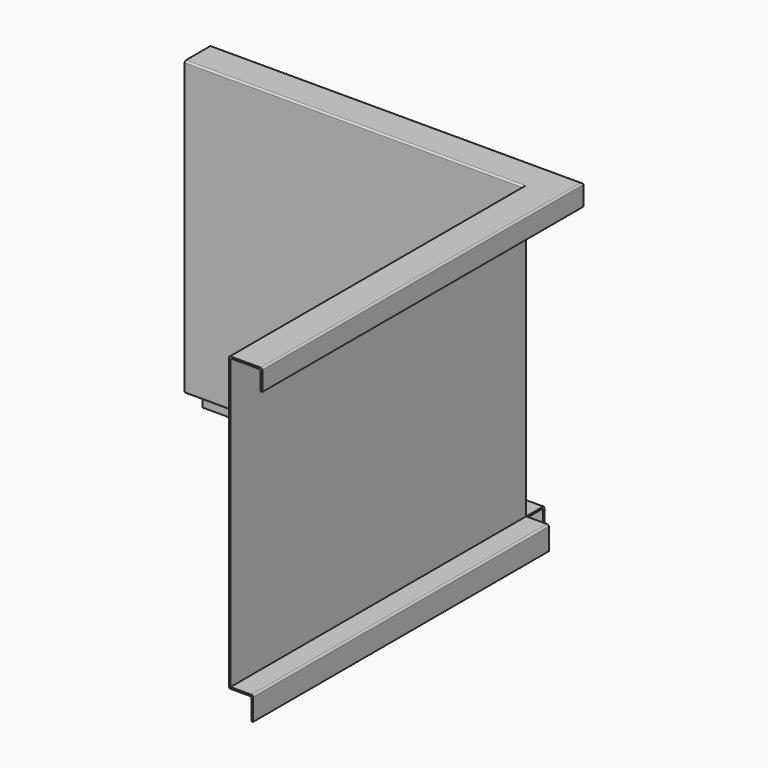
from build123d import *

# Parameters (mm, degrees)
F3_W         = 27
F3_H         = 27
F4_DEPTH     = 30
F5_T1_DEPTH  = 407
F5_T3_DEPTH  = 443
F5_T5_DEPTH  = 442
F5_T7_DEPTH  = 478
F5_T13_DEPTH = 447
F5_T17_DEPTH = 412
F5_T20_DEPTH = 417
F5_T22_DEPTH = 455
F5_T24_DEPTH = 410
F5_T26_DEPTH = 445
F5_T28_DEPTH = 490
F5_T30_DEPTH = 452
F5_T36_DEPTH = 415
F5_T40_DEPTH = 450
F5_T47_DEPTH = 415
F5_T51_DEPTH = 450


# Not quite as in the source:
# - a fillet or chamfer that OpenCascade refuses, or shapes differently, is made with other operations: its cross-section is extruded or revolved along the edge and cut away or added


with BuildPart() as f2:
    # F2: sweep along a path in F1
    with BuildLine(Plane.XY) as f2_path:
        Line((0, 0), (0, 440))
        Line((0, 440), (-405, 440))
    # F0 (on Front) → F2 (sweep)
    with BuildSketch(Plane.XZ):
        Polygon((38, -2), (38, -25), (40, -25), (40, 0), (0, 0), (0, -350), (27, -350), (27, -376), (29, -376), (29, -348), (2, -348), (2, -2), align=None)
    sweep(path=f2_path.line, transition=Transition.RIGHT)

    # F3 (on face) → F4 (cut)
    with BuildSketch(Plane.XY.offset(-348)):
        with Locations((15.5, 455.5)):
            Rectangle(F3_W, F3_H)
    extrude(amount=-F4_DEPTH, mode=Mode.SUBTRACT)

    # F5: fillet of radius 2 on 15 edges, made by hand

    # F5_s2 → F5_t1 (join)
    with BuildSketch(Plane.YZ.offset(-405)):
        with BuildLine():
            ThreePointArc((442, -346), (442.5857864376, -347.4142135624), (444, -348))
            Line((444, -348), (442, -348))
            Line((442, -348), (442, -346))
        make_face()
        with BuildLine():
            ThreePointArc((465, -350), (466.4142135624, -350.5857864376), (467, -352))
            Line((467, -352), (467, -350))
            Line((467, -350), (465, -350))
        make_face()
        with BuildLine():
            ThreePointArc((444, -2), (442.5857864376, -2.5857864376), (442, -4))
            Line((442, -4), (442, -2))
            Line((442, -2), (444, -2))
        make_face()
    extrude(amount=F5_T1_DEPTH)

    # F5_s4 → F5_t3 (join)
    with BuildSketch(Plane.YZ.offset(-405)):
        with BuildLine():
            ThreePointArc((476, -2), (477.4142135624, -2.5857864376), (478, -4))
            Line((478, -4), (478, -2))
            Line((478, -2), (476, -2))
        make_face()
    extrude(amount=F5_T3_DEPTH)

    # F5_s6 → F5_t5 (join)
    with BuildSketch(Plane.XZ.offset(-442)):
        with BuildLine():
            ThreePointArc((25, -350), (26.4142135624, -350.5857864376), (27, -352))
            Line((27, -352), (27, -350))
            Line((27, -350), (25, -350))
        make_face()
        with BuildLine():
            ThreePointArc((4, -2), (2.5857864376, -2.5857864376), (2, -4))
            Line((2, -4), (2, -2))
            Line((2, -2), (4, -2))
        make_face()
    extrude(amount=F5_T5_DEPTH)

    # F5_s8 → F5_t7 (join)
    with BuildSketch(Plane.XZ.offset(-478)):
        with BuildLine():
            ThreePointArc((38, -4), (37.4142135624, -2.5857864376), (36, -2))
            Line((36, -2), (38, -2))
            Line((38, -2), (38, -4))
        make_face()
    extrude(amount=F5_T7_DEPTH)


with BuildPart() as f5_tool11:
    # F5_s12 → F5_t13 (new body)
    with BuildSketch(Plane.XZ):
        with BuildLine():
            ThreePointArc((4, -2), (2.5857864376, -2.5857864376), (2, -4))
            Line((2, -4), (2, -2))
            Line((2, -2), (4, -2))
        make_face()
    extrude(amount=-F5_T13_DEPTH)

    split(bisect_by=Plane.XZ.offset(-442), keep=Keep.BOTTOM)


with BuildPart() as f5_tool15:
    # F5_s16 → F5_t17 (new body)
    with BuildSketch(Plane.YZ.offset(7)):
        with BuildLine():
            ThreePointArc((444, -2), (442.5857864376, -2.5857864376), (442, -4))
            Line((442, -4), (442, -2))
            Line((442, -2), (444, -2))
        make_face()
    extrude(amount=-F5_T17_DEPTH)

    split(bisect_by=Plane.YZ.offset(2), keep=Keep.TOP)


with BuildPart() as f5_tool11_1:
    add(f5_tool11.part)

    # F5_t19: intersect F5_tool15
    add(f5_tool15.part, mode=Mode.INTERSECT)


with BuildPart() as f2_1:
    add(f2.part)

    # F5_t9: union F5_tool11
    add(f5_tool11_1.part)

    # F5_s21 → F5_t20 (cut)
    with BuildSketch(Plane.YZ.offset(-410)):
        with BuildLine():
            ThreePointArc((467, -348), (468.4142135624, -348.5857864376), (469, -350))
            Line((469, -350), (469, -348))
            Line((469, -348), (467, -348))
        make_face()
    extrude(amount=F5_T20_DEPTH, mode=Mode.SUBTRACT)

    # F5_s23 → F5_t22 (cut)
    with BuildSketch(Plane.YZ.offset(-410)):
        with BuildLine():
            ThreePointArc((480, -2), (479.4142135624, -0.5857864376), (478, 0))
            Line((478, 0), (480, 0))
            Line((480, 0), (480, -2))
        make_face()
    extrude(amount=F5_T22_DEPTH, mode=Mode.SUBTRACT)

    # F5_s25 → F5_t24 (cut)
    with BuildSketch(Plane.YZ.offset(-410)):
        with BuildLine():
            ThreePointArc((440, -2), (440.5857864376, -0.5857864376), (442, 0))
            Line((442, 0), (440, 0))
            Line((440, 0), (440, -2))
        make_face()
        with BuildLine():
            ThreePointArc((440, -348), (440.5857864376, -349.4142135624), (442, -350))
            Line((442, -350), (440, -350))
            Line((440, -350), (440, -348))
        make_face()
    extrude(amount=F5_T24_DEPTH, mode=Mode.SUBTRACT)

    # F5_s27 → F5_t26 (cut)
    with BuildSketch(Plane.XZ.offset(-440)):
        with BuildLine():
            ThreePointArc((0, -2), (0.5857864376, -0.5857864376), (2, 0))
            Line((2, 0), (0, 0))
            Line((0, 0), (0, -2))
        make_face()
        with BuildLine():
            ThreePointArc((2, -350), (0.5857864376, -349.4142135624), (0, -348))
            Line((0, -348), (0, -350))
            Line((0, -350), (2, -350))
        make_face()
    extrude(amount=F5_T26_DEPTH, mode=Mode.SUBTRACT)

    # F5_s29 → F5_t28 (cut)
    with BuildSketch(Plane.XZ.offset(-485)):
        with BuildLine():
            ThreePointArc((38, 0), (39.4142135624, -0.5857864376), (40, -2))
            Line((40, -2), (40, 0))
            Line((40, 0), (38, 0))
        make_face()
    extrude(amount=F5_T28_DEPTH, mode=Mode.SUBTRACT)

    # F5_s31 → F5_t30 (cut)
    with BuildSketch(Plane.XZ.offset(-447)):
        with BuildLine():
            ThreePointArc((27, -348), (28.4142135624, -348.5857864376), (29, -350))
            Line((29, -350), (29, -348))
            Line((29, -348), (27, -348))
        make_face()
    extrude(amount=F5_T30_DEPTH, mode=Mode.SUBTRACT)


with BuildPart() as f5_tool34:
    # F5_s35 → F5_t36 (new body)
    with BuildSketch(Plane.YZ.offset(5)):
        with BuildLine():
            ThreePointArc((440, -2), (440.5857864376, -0.5857864376), (442, 0))
            Line((442, 0), (440, 0))
            Line((440, 0), (440, -2))
        make_face()
    extrude(amount=-F5_T36_DEPTH)

    split(bisect_by=Plane.YZ, keep=Keep.TOP)


with BuildPart() as f5_tool38:
    # F5_s39 → F5_t40 (new body)
    with BuildSketch(Plane.XZ.offset(5)):
        with BuildLine():
            ThreePointArc((0, -2), (0.5857864376, -0.5857864376), (2, 0))
            Line((2, 0), (0, 0))
            Line((0, 0), (0, -2))
        make_face()
    extrude(amount=-F5_T40_DEPTH)

    split(bisect_by=Plane.XZ.offset(-440), keep=Keep.BOTTOM)


with BuildPart() as f5_tool34_1:
    add(f5_tool34.part)

    # F5_t42: intersect F5_tool38
    add(f5_tool38.part, mode=Mode.INTERSECT)


with BuildPart() as f2_2:
    add(f2_1.part)

    # F5_t32: cut F5_tool34
    add(f5_tool34_1.part, mode=Mode.SUBTRACT)


with BuildPart() as f5_tool45:
    # F5_s46 → F5_t47 (new body)
    with BuildSketch(Plane.YZ.offset(5)):
        with BuildLine():
            ThreePointArc((440, -348), (440.5857864376, -349.4142135624), (442, -350))
            Line((442, -350), (440, -350))
            Line((440, -350), (440, -348))
        make_face()
    extrude(amount=-F5_T47_DEPTH)

    split(bisect_by=Plane.YZ, keep=Keep.TOP)


with BuildPart() as f5_tool49:
    # F5_s50 → F5_t51 (new body)
    with BuildSketch(Plane.XZ.offset(5)):
        with BuildLine():
            ThreePointArc((2, -350), (0.5857864376, -349.4142135624), (0, -348))
            Line((0, -348), (0, -350))
            Line((0, -350), (2, -350))
        make_face()
    extrude(amount=-F5_T51_DEPTH)

    split(bisect_by=Plane.XZ.offset(-440), keep=Keep.BOTTOM)


with BuildPart() as f5_tool45_1:
    add(f5_tool45.part)

    # F5_t53: intersect F5_tool49
    add(f5_tool49.part, mode=Mode.INTERSECT)


with BuildPart() as f2_3:
    add(f2_2.part)

    # F5_t43: cut F5_tool45
    add(f5_tool45_1.part, mode=Mode.SUBTRACT)


solid = f2_3.part
